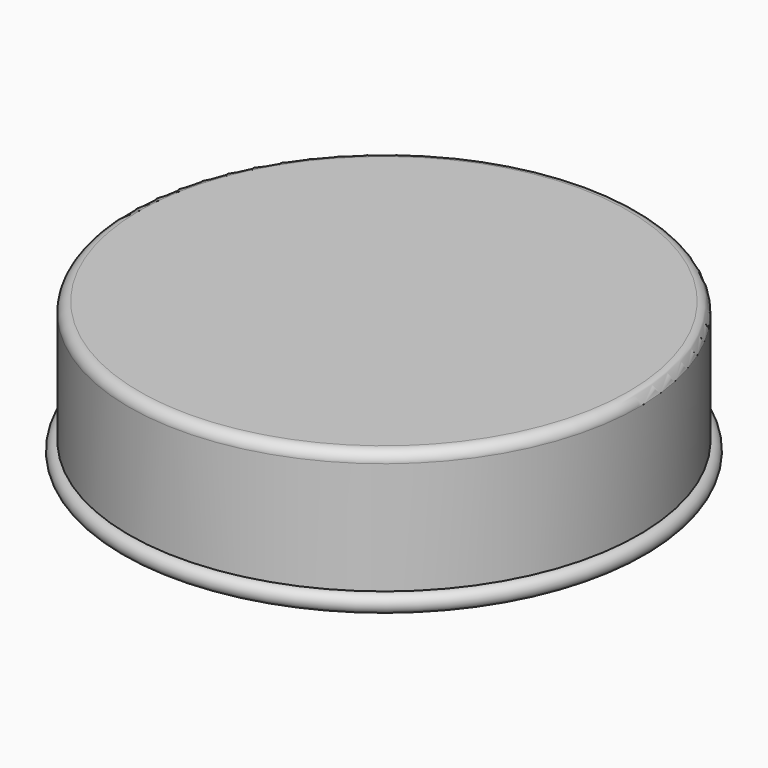
from build123d import *


# Not quite as in the source:
# - a feature names something its author has since deleted; it is built from what else it names


with BuildPart() as f1:
    # F0 (on Right) → F1 (revolve)
    with BuildSketch(Plane.YZ):
        with BuildLine():
            Line((21.5, 4), (21.5, 0))
            Line((21.5, 0), (24.5, 0))
            Line((24.5, 0), (24.5, 1.7079167301))
            Line((24.5, 1.7079167301), (24.5, 12.5))
            ThreePointArc((24.5, 12.5), (24.2071067812, 13.2071067812), (23.5, 13.5))
            Line((23.5, 13.5), (0, 13.5))
            Line((0, 13.5), (0, 12.5))
            Line((0, 12.5), (22.5, 12.5))
            Line((22.5, 12.5), (23.5, 12.5))
            Line((23.5, 12.5), (23.5, 7.5))
            Line((23.5, 7.5), (22.5, 7.5))
            Line((22.5, 7.5), (22.5, 4))
            Line((22.5, 4), (21.5, 4))
        make_face()
        with BuildLine():
            Line((24.5, 1.7079167301), (24.5, 0))
            ThreePointArc((24.5, 0), (25.353958365, 0.853958365), (24.5, 1.7079167301))
        make_face()
    revolve(axis=Axis((0, 0, 6.75), (0, 0, 1)))


solid = f1.part
